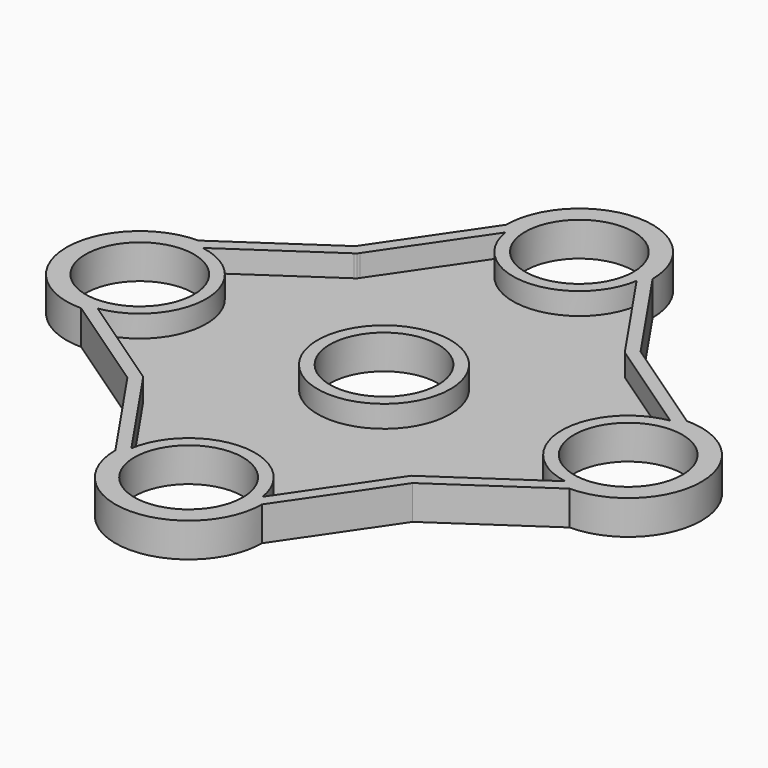
from build123d import *

# Parameters (mm, degrees)
F0_R        = 11.1
F1_DEPTH    = 3.5
F2_T        = 2.5
F2_T3_DEPTH = 12


# Not quite as in the source:
# - a shell that OpenCascade refuses in one call is made with other operations: the cavity is built on its own and cut out


with BuildPart() as f1:
    # F0 (on Top) → F1 (new body, symmetric)
    with BuildSketch(Plane.XY):
        with BuildLine():
            Line((29.2040910572, 29.1611850262), (15, 50))
            ThreePointArc((15, 50), (0, 35), (-15, 50))
            Line((-15, 50), (-29.2040910572, 29.1611850262))
            Line((-29.2040910572, 29.1611850262), (-50, 15))
            ThreePointArc((-50, 15), (-39.3933982822, 10.6066017178), (-35, 0))
            ThreePointArc((-35, 0), (-39.3933982822, -10.6066017178), (-50, -15))
            Line((-50, -15), (-29.2040910572, -29.1611850262))
            Line((-29.2040910572, -29.1611850262), (-15, -50))
            ThreePointArc((-15, -50), (0, -35), (15, -50))
            Line((15, -50), (29.2040910572, -29.1611850262))
            Line((29.2040910572, -29.1611850262), (50, -15))
            ThreePointArc((50, -15), (35, 0), (50, 15))
            Line((50, 15), (29.2040910572, 29.1611850262))
        make_face()
        Circle(F0_R, mode=Mode.SUBTRACT)
        with BuildLine():
            ThreePointArc((-15, 50), (0, 35), (15, 50))
            ThreePointArc((15, 50), (0, 65), (-15, 50))
        make_face()
        with Locations((0, 50)):
            Circle(F0_R, mode=Mode.SUBTRACT)
        with BuildLine():
            ThreePointArc((65, 0), (60.6066017178, 10.6066017178), (50, 15))
            ThreePointArc((50, 15), (35, 0), (50, -15))
            ThreePointArc((50, -15), (60.6066017178, -10.6066017178), (65, 0))
        make_face()
        with Locations((50, 0)):
            Circle(F0_R, mode=Mode.SUBTRACT)
        with BuildLine():
            ThreePointArc((-15, -50), (0, -65), (15, -50))
            ThreePointArc((15, -50), (0, -35), (-15, -50))
        make_face()
        with Locations((0, -50)):
            Circle(F0_R, mode=Mode.SUBTRACT)
        with BuildLine():
            ThreePointArc((-35, 0), (-39.3933982822, 10.6066017178), (-50, 15))
            ThreePointArc((-50, 15), (-65, 0), (-50, -15))
            ThreePointArc((-50, -15), (-39.3933982822, -10.6066017178), (-35, 0))
        make_face()
        with Locations((-50, 0)):
            Circle(F0_R, mode=Mode.SUBTRACT)
    extrude(amount=F1_DEPTH, both=True)

    # F2: shell of thickness 2.5, made by hand


with BuildPart() as f2_core1:
    # F2_t2: copy of F1
    add(f1.part)

    # the walls: a layer under each face that stays
    f2_faces = [f2_core1.faces().sort_by_distance(p)[0] for p in [
        (39.6020455286, -22.0805925131, 0),
        (22.1020455286, -39.5805925131, 0),
        (0, -65, 0),
        (-22.1020455286, -39.5805925131, 0),
        (-39.6020455286, -22.0805925131, 0),
        (-65, 0, 0),
        (-39.6020455286, 22.0805925131, 0),
        (-22.1020455286, 39.5805925131, 0),
        (0, 65, 0),
        (22.1020455286, 39.5805925131, 0),
        (39.6020455286, 22.0805925131, 0),
        (-61.1, 0, 0),
        (-11.1, -50, 0),
        (38.9, 0, 0),
        (-11.1, 50, 0),
        (-11.1, 0, 0),
        (65, 0, 0),
        (-37.1428571429, -18.5714285714, -3.5),
    ]]
    thicken(f2_faces, amount=-F2_T, mode=Mode.SUBTRACT)

    # F2_s4 → F2_t3 (cut)
    with BuildSketch(Plane.XY.offset(-6)):
        Polygon((50.0140713144, -15.0456639326), (48.5928685595, -12.933606739), (49.2296264469, -12.5), (50, -12.5), align=None)
        Polygon((29.2388199891, -29.1959295426), (27.7969596167, -27.0947917651), (27.4052462259, -27.3615329699), (27.1383293075, -27.753126649), align=None)
        Polygon((15.0456576175, -50.0140805838), (12.9342382503, -48.5919416228), (12.5, -49.2290123454), (12.5, -50), align=None)
        Polygon((-15.0456576175, -50.0140805838), (-12.5, -50), (-12.5, -49.2290123454), (-12.9342382503, -48.5919416228), align=None)
        Polygon((-29.2388199891, -29.1959295426), (-27.1383293075, -27.753126649), (-27.4052462259, -27.3615329699), (-27.7969596167, -27.0947917651), align=None)
        Polygon((-50.0140713144, -15.0456639326), (-48.5928685595, -12.933606739), (-49.2296264469, -12.5), (-50, -12.5), align=None)
        Polygon((-50.0140713144, 15.0456639326), (-50, 12.5), (-49.2296264469, 12.5), (-48.5928685595, 12.933606739), align=None)
        Polygon((-29.2388199891, 29.1959295426), (-27.7969596167, 27.0947917651), (-27.4052462259, 27.3615329699), (-27.1383293075, 27.753126649), align=None)
        Polygon((-15.0456576175, 50.0140805838), (-12.9342382503, 48.5919416228), (-12.5, 49.2290123454), (-12.5, 50), align=None)
        Polygon((15.0456576175, 50.0140805838), (12.5, 50), (12.5, 49.2290123454), (12.9342382503, 48.5919416228), align=None)
        Polygon((29.2388199891, 29.1959295426), (27.1383293075, 27.753126649), (27.4052462259, 27.3615329699), (27.7969596167, 27.0947917651), align=None)
        Polygon((50.0140713144, 15.0456639326), (48.5928685595, 12.933606739), (49.2296264469, 12.5), (50, 12.5), align=None)
    extrude(amount=F2_T3_DEPTH, mode=Mode.SUBTRACT)


with BuildPart() as f1_1:
    add(f1.part)

    # what is left inside the walls is the cavity
    f2_cavity = [f2_core1.part.solids().sort_by_distance(p)[0] for p in [
        (0, -15.95435, 3.475),
    ]]
    add(f2_cavity, mode=Mode.SUBTRACT)


solid = f1_1.part
